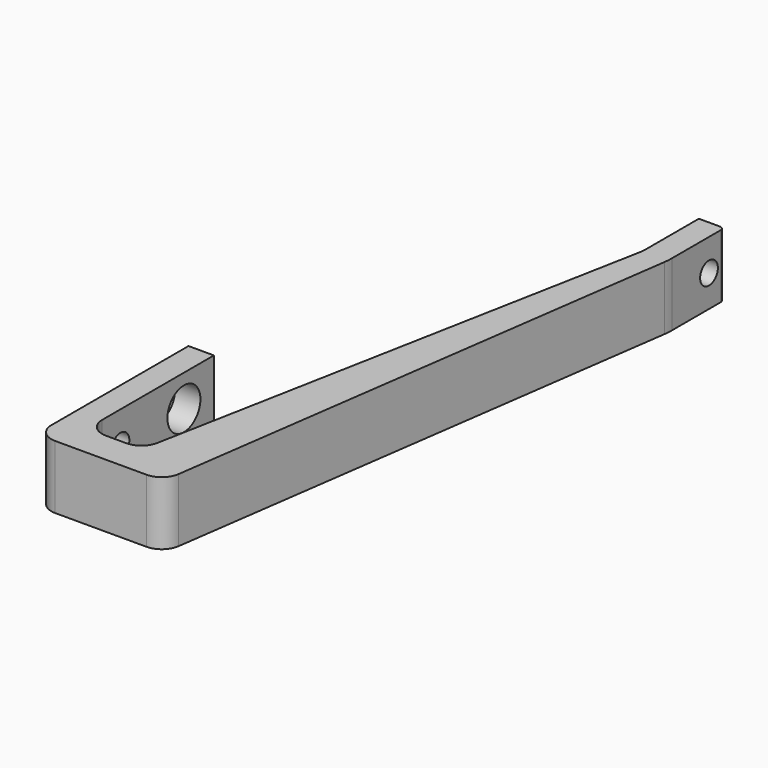
from build123d import *

# Parameters (mm, degrees)
F0_W     = 4
F0_H     = 25
F1_DEPTH = 10
F2_R     = 3
F3_R     = 10
F4_R     = 1.75
F5_DEPTH = 5
F6_R     = 3.25
F6_R_2   = 1.75
F7_DEPTH = 6
F8_R     = 0.7


# Not quite as in the source:
# - a feature names something its author has since deleted; it is built from what else it names


with BuildPart() as f1:
    # F0 (on Top) → F1 (new body)
    with BuildSketch(Plane.XY):
        with Locations((2, 17.5)):
            Rectangle(F0_W, F0_H)
        Polygon((0, 5), (0, 0), (20, 0), (31.84, 84.7), (31.84, 95.7), (27.84, 95.7), (27.84, 84.7), (12.6761412248, 5), (4, 5), align=None)
    extrude(amount=F1_DEPTH)

    # F2
    f2_edges = [f1.edges().sort_by_distance(p)[0] for p in [
        (12.676141, 5, 5),
        (4, 5, 5),
        (0, 0, 5),
        (20, 0, 5),
    ]]
    fillet(f2_edges, radius=F2_R)

    # F3
    f3_edges = [f1.edges().sort_by_distance(p)[0] for p in [
        (27.84, 84.7, 5),
        (31.84, 84.7, 5),
    ]]
    fillet(f3_edges, radius=F3_R)

    # F4 (on face) → F5 (cut)
    with BuildSketch(Plane.YZ.offset(31.84)):
        with Locations((92.7, 5)):
            Circle(F4_R)
    extrude(amount=-F5_DEPTH, mode=Mode.SUBTRACT)

    # F6 (on face) → F7 (cut)
    with BuildSketch(Plane(origin=(0, 0, 0), x_dir=(0, -1, 0), z_dir=(-1, 0, 0))):
        with Locations((-24.1, 5)):
            Circle(F6_R)
        with Locations((-11.6, 5)):
            Circle(F6_R_2)
    extrude(amount=-F7_DEPTH, mode=Mode.SUBTRACT)

    # F8
    f8_edges = [f1.edges().sort_by_distance(p)[0] for p in [
        (31.84, 95.7, 5),
    ]]
    fillet(f8_edges, radius=F8_R)


solid = f1.part
